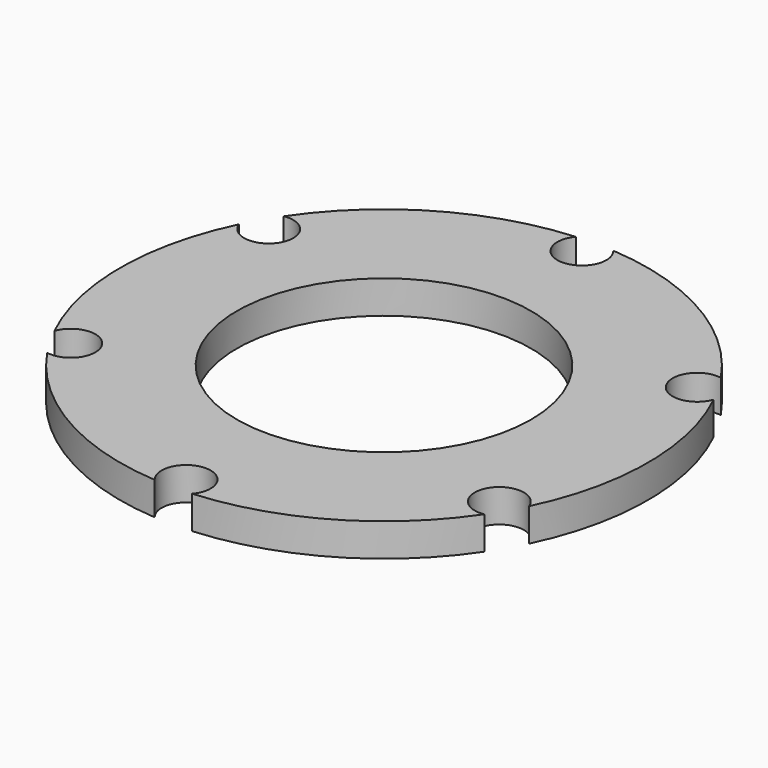
from build123d import *

# Parameters (mm, degrees)
F0_R            = 25.4
F0_R_2          = 14.1605
F1_DEPTH        = 3.175
F2_R            = 2.3622
F3_DEPTH        = 3.176
F3_COPIES_COUNT = 6


# Not quite as in the source:
# - a pattern or mirror of a feature is missing from the dataset's text; its kind, count and spacing are read off the source's solid


with BuildPart() as f1:
    # F0 (on Top) → F1 (new body)
    with BuildSketch(Plane.XY):
        Circle(F0_R)
        Circle(F0_R_2, mode=Mode.SUBTRACT)
    extrude(amount=F1_DEPTH)

    # F2 (on face) → F3 (cut, through all)
    with BuildSketch(Plane.XY.offset(3.175)):
        with Locations((0, 23.8125)):
            Circle(F2_R)
    f3 = extrude(amount=-F3_DEPTH, mode=Mode.SUBTRACT)

    # F3_copies: F3 ×6 about axis
    f3_copies_axis = Axis((0, 0, 0), (0, 0, 1))
    for i in range(1, F3_COPIES_COUNT):
        add(f3.rotate(f3_copies_axis, i * 360 / F3_COPIES_COUNT), mode=Mode.SUBTRACT)


solid = f1.part
